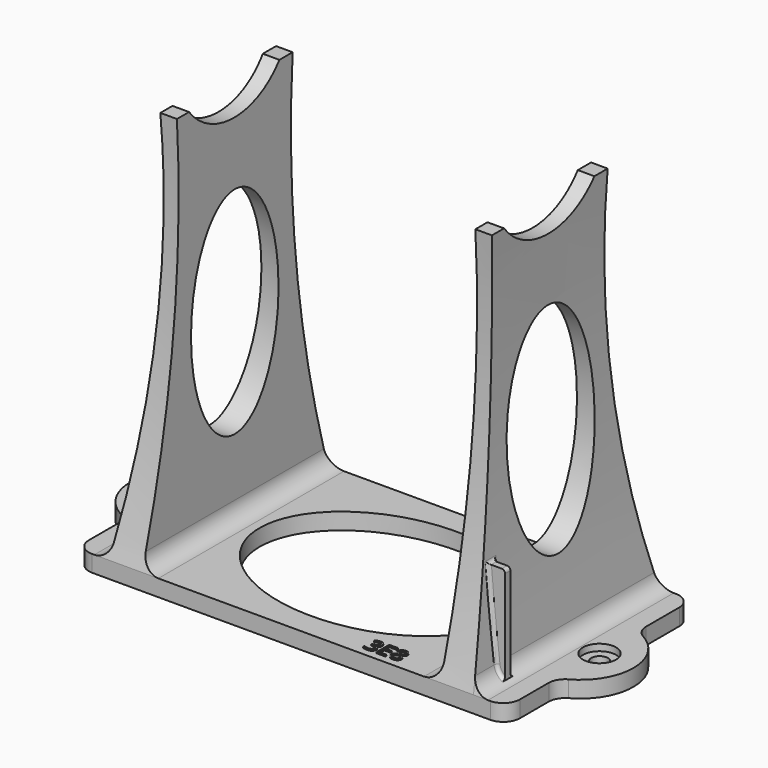
from build123d import *

# Parameters (mm, degrees)
F1_DEPTH       = 35
F3_DEPTH       = 65.001
F3_DEPTH_BACK  = 65.001
F5_DEPTH       = 5.001
F6_DEPTH       = 5
F7_D           = 5
F7_CBORE_D     = 10
F7_CBORE_DEPTH = 2
F8_T1_DEPTH    = 5
F8_T6_DEPTH    = 70
F8_S7_R        = 330
F8_T8_DEPTH    = 37
F8_S9_R        = 330
F8_T10_DEPTH   = 37
F8_T14_DEPTH   = 70
F8_S15_R       = 330
F8_T16_DEPTH   = 37
F8_S17_R       = 330
F8_T18_DEPTH   = 37
F8_T22_DEPTH   = 70
F8_S23_R       = 330
F8_T24_DEPTH   = 37
F8_S25_R       = 330
F8_T26_DEPTH   = 37
F8_T30_DEPTH   = 70
F8_S31_R       = 330
F8_T32_DEPTH   = 37
F8_S33_R       = 330
F8_T34_DEPTH   = 37
F8_T35_DEPTH   = 30.0048285071
F9_TEXT_SIZE   = 6.7275793602
F10_DEPTH      = 0.3
F12_W          = 2
F12_H          = 30
F13_DEPTH      = 5.5
F14_R          = 1


# Not quite as in the source:
# - a fillet or chamfer that OpenCascade refuses, or shapes differently, is made with other operations: its cross-section is extruded or revolved along the edge and cut away or added
# - Text() gives the source's letters only with a copy of the font that has no kerning and outlines rounded to 1/6400 em; it was checked with that copy


with BuildPart() as f1:
    # F0 (on Front) → F1 (new body, symmetric)
    with BuildSketch(Plane.XZ):
        with BuildLine():
            Line((-65, 5), (-65, 0))
            Line((-65, 0), (65, 0))
            Line((65, 0), (65, 5))
            Line((65, 5), (55, 5))
            ThreePointArc((55, 5), (50.1321532001, 62.3970501391), (50, 120))
            Line((50, 120), (45, 120))
            Line((45, 120), (45, 5))
            Line((45, 5), (0, 5))
            Line((0, 5), (-45, 5))
            Line((-45, 5), (-45, 120))
            Line((-45, 120), (-50, 120))
            ThreePointArc((-50, 120), (-50.1321532001, 62.3970501391), (-55, 5))
            Line((-55, 5), (-65, 5))
        make_face()
    extrude(amount=F1_DEPTH, both=True)

    # F2 (on Right) → F3 (cut, two sides)
    with BuildSketch(Plane.YZ) as f3_sk:
        with BuildLine():
            Line((21.2042803188, 133.2788269271), (-21.6306972347, 132.7176760803))
            ThreePointArc((-21.6306972347, 132.7176760803), (-6.9407226467, 112.6628611482), (16.8112740868, 120))
            ThreePointArc((16.8112740868, 120), (20.1221818976, 126.270737315), (21.2042803188, 133.2788269271))
        make_face()
        with BuildLine():
            Line((35, 120), (21.8112740868, 120))
            ThreePointArc((21.8112740868, 120), (23.3239482349, 61.9172086881), (35, 5))
            Line((35, 5), (35, 120))
        make_face()
        with BuildLine():
            add(Edge.make_bspline(
                [(0, 92.5), (-28.5788383249, 92.5), (-14.2894191624, 43.75), (0, -5), (14.2894191624, 43.75), (28.5788383249, 92.5), (0, 92.5)],
                knots=[0, 0, 0, 2.0943951024, 2.0943951024, 4.1887902048, 4.1887902048, 6.2831853072, 6.2831853072, 6.2831853072], degree=2, weights=[1, 0.5, 1, 0.5, 1, 0.5, 1]))
        make_face()
        with BuildLine():
            ThreePointArc((-35, 5), (-23.3239482349, 61.9172086881), (-21.8112740868, 120))
            Line((-21.8112740868, 120), (-35, 120))
            Line((-35, 120), (-35, 5))
        make_face()
    extrude(amount=-F3_DEPTH, mode=Mode.SUBTRACT)
    extrude(f3_sk.sketch, amount=F3_DEPTH_BACK, mode=Mode.SUBTRACT)

    # F4 (on face) → F5 (cut, through all)
    with BuildSketch(Plane.XY.offset(5)):
        with BuildLine():
            add(Edge.make_bspline(
                [(37.5, 0), (37.5, 47.6313972081), (-18.75, 23.8156986041), (-75, 0), (-18.75, -23.8156986041), (37.5, -47.6313972081), (37.5, 0)],
                knots=[0, 0, 0, 2.0943951024, 2.0943951024, 4.1887902048, 4.1887902048, 6.2831853072, 6.2831853072, 6.2831853072], degree=2, weights=[1, 0.5, 1, 0.5, 1, 0.5, 1]))
        make_face()
    extrude(amount=-F5_DEPTH, mode=Mode.SUBTRACT)

    # F4 (on face) → F6 (join)
    with BuildSketch(Plane.XY.offset(5)):
        with BuildLine():
            Line((65, 14.3543907626), (65, -15.9574002028))
            ThreePointArc((65, -15.9574002028), (75.8717613044, -0.8015047201), (65, 14.3543907626))
        make_face()
        with BuildLine():
            ThreePointArc((-65, 14.3543907626), (-75.8717613044, -0.8015047201), (-65, -15.9574002028))
            Line((-65, -15.9574002028), (-65, 14.3543907626))
        make_face()
    extrude(amount=-F6_DEPTH)

    # F7 (through all)
    with Locations(Plane.XY.offset(5)):
        with Locations((65, 0), (-65, -0.8015047201)):
            CounterBoreHole(F7_D / 2, F7_CBORE_D / 2, F7_CBORE_DEPTH)

    # F8: fillet of radius 5 on 12 edges, made by hand

    # F8_s2 → F8_t1 (join)
    with BuildSketch(Plane.XY):
        with BuildLine():
            ThreePointArc((64.9996, -19.1986916005), (65.6953355382, -16.6538385791), (67.58900558, -14.8169012878))
            Line((67.58900558, -14.8169012878), (67.3477327338, -14.3787222566))
            ThreePointArc((67.3477327338, -14.3787222566), (66.118244301, -14.9868786908), (64.8396741415, -15.4835763232))
            Line((64.8396741415, -15.4835763232), (64.4997865958, -15.9574002028))
            ThreePointArc((64.4997865958, -15.9574002028), (64.4997865958, -17.5780459016), (64.4993865958, -19.1986916005))
            Line((64.4993865958, -19.1986916005), (64.9996, -19.1986916005))
        make_face()
        with BuildLine():
            ThreePointArc((-67.58900558, -14.8169012878), (-65.6953355382, -16.6538385791), (-64.9996, -19.1986916005))
            Line((-64.9996, -19.1986916005), (-64.4993865958, -19.1986916005))
            ThreePointArc((-64.4993865958, -19.1986916005), (-64.4997865958, -17.5780459016), (-64.4997865958, -15.9574002028))
            Line((-64.4997865958, -15.9574002028), (-64.8396741415, -15.4835763232))
            ThreePointArc((-64.8396741415, -15.4835763232), (-66.118244301, -14.9868786908), (-67.3477327338, -14.3787222566))
            Line((-67.3477327338, -14.3787222566), (-67.58900558, -14.8169012878))
        make_face()
        with BuildLine():
            ThreePointArc((-64.9996, 17.5956821603), (-65.6953355382, 15.0508291389), (-67.58900558, 13.2138918476))
            Line((-67.58900558, 13.2138918476), (-67.3477327338, 12.7757128164))
            ThreePointArc((-67.3477327338, 12.7757128164), (-66.118244301, 13.3838692506), (-64.8396741415, 13.880566883))
            Line((-64.8396741415, 13.880566883), (-64.4997865958, 14.3543907626))
            ThreePointArc((-64.4997865958, 14.3543907626), (-64.4997865958, 15.9750364614), (-64.4993865958, 17.5956821603))
            Line((-64.4993865958, 17.5956821603), (-64.9996, 17.5956821603))
        make_face()
        with BuildLine():
            ThreePointArc((64.9996, 17.5956821603), (65.6953355382, 15.0508291389), (67.58900558, 13.2138918476))
            Line((67.58900558, 13.2138918476), (67.3477327338, 12.7757128164))
            ThreePointArc((67.3477327338, 12.7757128164), (66.118244301, 13.3838692506), (64.8396741415, 13.880566883))
            Line((64.8396741415, 13.880566883), (64.4997865958, 14.3543907626))
            ThreePointArc((64.4997865958, 14.3543907626), (64.4997865958, 15.9750364614), (64.4993865958, 17.5956821603))
            Line((64.4993865958, 17.5956821603), (64.9996, 17.5956821603))
        make_face()
    extrude(amount=F8_T1_DEPTH)


with BuildPart() as f8_tool4:
    # F8_s5 → F8_t6 (new body)
    with BuildSketch(Plane.XZ.offset(-35)):
        with BuildLine():
            ThreePointArc((59.4227881967, 4.9996), (56.1034800472, 6.2597833835), (54.4568111339, 9.4053119944))
            Line((54.4568111339, 9.4053119944), (53.9602134276, 9.3457231014))
            ThreePointArc((53.9602134276, 9.3457231014), (54.2287059943, 7.1410871793), (54.5037901262, 4.937263414))
            Line((54.5037901262, 4.937263414), (55, 4.4998399076))
            ThreePointArc((55, 4.4998399076), (57.2113940983, 4.4998399076), (59.4227881967, 4.4994399076))
            Line((59.4227881967, 4.4994399076), (59.4227881967, 4.9996))
        make_face()
    extrude(amount=F8_T6_DEPTH)

    # F8_s7 → F8_t8 (cut, symmetric)
    with BuildSketch(Plane.YZ.offset(56.7)):
        with Locations((351.1749527639, 99.5166612019)):
            Circle(F8_S7_R)
    extrude(amount=F8_T8_DEPTH, both=True, mode=Mode.SUBTRACT)

    # F8_s9 → F8_t10 (cut, symmetric)
    with BuildSketch(Plane.YZ.offset(56.7)):
        with Locations((-351.1749527639, 99.5166612019)):
            Circle(F8_S9_R)
    extrude(amount=F8_T10_DEPTH, both=True, mode=Mode.SUBTRACT)


with BuildPart() as f1_1:
    add(f1.part)

    # F8_t3: union F8_tool4
    add(f8_tool4.part)


with BuildPart() as f8_tool12:
    # F8_s13 → F8_t14 (new body)
    with BuildSketch(Plane.XZ.offset(35)):
        with BuildLine():
            ThreePointArc((-59.4227881967, 4.9996), (-56.1034800472, 6.2597833835), (-54.4568111339, 9.4053119944))
            Line((-54.4568111339, 9.4053119944), (-53.9602134276, 9.3457231014))
            ThreePointArc((-53.9602134276, 9.3457231014), (-54.2287059943, 7.1410871793), (-54.5037901262, 4.937263414))
            Line((-54.5037901262, 4.937263414), (-55, 4.4998399076))
            ThreePointArc((-55, 4.4998399076), (-57.2113940983, 4.4998399076), (-59.4227881967, 4.4994399076))
            Line((-59.4227881967, 4.4994399076), (-59.4227881967, 4.9996))
        make_face()
    extrude(amount=-F8_T14_DEPTH)

    # F8_s15 → F8_t16 (cut, symmetric)
    with BuildSketch(Plane.YZ.offset(-56.7)):
        with Locations((351.1749527639, 99.5166612019)):
            Circle(F8_S15_R)
    extrude(amount=F8_T16_DEPTH, both=True, mode=Mode.SUBTRACT)

    # F8_s17 → F8_t18 (cut, symmetric)
    with BuildSketch(Plane.YZ.offset(-56.7)):
        with Locations((-351.1749527639, 99.5166612019)):
            Circle(F8_S17_R)
    extrude(amount=F8_T18_DEPTH, both=True, mode=Mode.SUBTRACT)


with BuildPart() as f1_2:
    add(f1_1.part)

    # F8_t11: union F8_tool12
    add(f8_tool12.part)


with BuildPart() as f8_tool20:
    # F8_s21 → F8_t22 (new body)
    with BuildSketch(Plane.XZ.offset(-35)):
        with BuildLine():
            ThreePointArc((39.9990343146, 4.9996), (43.5355339059, 6.4644660941), (45.0004, 10.0009656854))
            Line((45.0004, 10.0009656854), (45.5005365685, 10.0009656854))
            ThreePointArc((45.5005365685, 10.0009656854), (45.5001365685, 7.5004828427), (45.5001365685, 5))
            Line((45.5001365685, 5), (45, 4.4998634315))
            ThreePointArc((45, 4.4998634315), (42.4995171573, 4.4998634315), (39.9990343146, 4.4994634315))
            Line((39.9990343146, 4.4994634315), (39.9990343146, 4.9996))
        make_face()
    extrude(amount=F8_T22_DEPTH)

    # F8_s23 → F8_t24 (cut, symmetric)
    with BuildSketch(Plane.YZ.offset(42.7)):
        with Locations((351.1749527639, 99.5166612019)):
            Circle(F8_S23_R)
    extrude(amount=F8_T24_DEPTH, both=True, mode=Mode.SUBTRACT)

    # F8_s25 → F8_t26 (cut, symmetric)
    with BuildSketch(Plane.YZ.offset(42.7)):
        with Locations((-351.1749527639, 99.5166612019)):
            Circle(F8_S25_R)
    extrude(amount=F8_T26_DEPTH, both=True, mode=Mode.SUBTRACT)


with BuildPart() as f1_3:
    add(f1_2.part)

    # F8_t19: union F8_tool20
    add(f8_tool20.part)


with BuildPart() as f8_tool28:
    # F8_s29 → F8_t30 (new body)
    with BuildSketch(Plane.XZ.offset(-35)):
        with BuildLine():
            ThreePointArc((-39.9990343146, 4.9996), (-43.5355339059, 6.4644660941), (-45.0004, 10.0009656854))
            Line((-45.0004, 10.0009656854), (-45.5005365685, 10.0009656854))
            ThreePointArc((-45.5005365685, 10.0009656854), (-45.5001365685, 7.5004828427), (-45.5001365685, 5))
            Line((-45.5001365685, 5), (-45, 4.4998634315))
            ThreePointArc((-45, 4.4998634315), (-42.4995171573, 4.4998634315), (-39.9990343146, 4.4994634315))
            Line((-39.9990343146, 4.4994634315), (-39.9990343146, 4.9996))
        make_face()
    extrude(amount=F8_T30_DEPTH)

    # F8_s31 → F8_t32 (cut, symmetric)
    with BuildSketch(Plane.YZ.offset(-42.7)):
        with Locations((351.1749527639, 99.5166612019)):
            Circle(F8_S31_R)
    extrude(amount=F8_T32_DEPTH, both=True, mode=Mode.SUBTRACT)

    # F8_s33 → F8_t34 (cut, symmetric)
    with BuildSketch(Plane.YZ.offset(-42.7)):
        with Locations((-351.1749527639, 99.5166612019)):
            Circle(F8_S33_R)
    extrude(amount=F8_T34_DEPTH, both=True, mode=Mode.SUBTRACT)


with BuildPart() as f1_4:
    add(f1_3.part)

    # F8_t27: union F8_tool28
    add(f8_tool28.part)

    # F8_s36 → F8_t35 (cut)
    with BuildSketch(Plane.XY.offset(-12.5024142536)):
        with BuildLine():
            ThreePointArc((59.9990343146, 35.0004), (63.5355339059, 33.5355339059), (65.0004, 29.9990343146))
            Line((65.0004, 29.9990343146), (65.5005365685, 29.9990343146))
            ThreePointArc((65.5005365685, 29.9990343146), (65.5001365685, 32.4995171573), (65.5001365685, 35))
            Line((65.5001365685, 35), (65, 35.5001365685))
            ThreePointArc((65, 35.5001365685), (62.4995171573, 35.5001365685), (59.9990343146, 35.5005365685))
            Line((59.9990343146, 35.5005365685), (59.9990343146, 35.0004))
        make_face()
        with BuildLine():
            ThreePointArc((-59.9990343146, 35.0004), (-63.5355339059, 33.5355339059), (-65.0004, 29.9990343146))
            Line((-65.0004, 29.9990343146), (-65.5005365685, 29.9990343146))
            ThreePointArc((-65.5005365685, 29.9990343146), (-65.5001365685, 32.4995171573), (-65.5001365685, 35))
            Line((-65.5001365685, 35), (-65, 35.5001365685))
            ThreePointArc((-65, 35.5001365685), (-62.4995171573, 35.5001365685), (-59.9990343146, 35.5005365685))
            Line((-59.9990343146, 35.5005365685), (-59.9990343146, 35.0004))
        make_face()
        with BuildLine():
            ThreePointArc((-59.9990343146, -35.0004), (-63.5355339059, -33.5355339059), (-65.0004, -29.9990343146))
            Line((-65.0004, -29.9990343146), (-65.5005365685, -29.9990343146))
            ThreePointArc((-65.5005365685, -29.9990343146), (-65.5001365685, -32.4995171573), (-65.5001365685, -35))
            Line((-65.5001365685, -35), (-65, -35.5001365685))
            ThreePointArc((-65, -35.5001365685), (-62.4995171573, -35.5001365685), (-59.9990343146, -35.5005365685))
            Line((-59.9990343146, -35.5005365685), (-59.9990343146, -35.0004))
        make_face()
        with BuildLine():
            ThreePointArc((59.9990343146, -35.0004), (63.5355339059, -33.5355339059), (65.0004, -29.9990343146))
            Line((65.0004, -29.9990343146), (65.5005365685, -29.9990343146))
            ThreePointArc((65.5005365685, -29.9990343146), (65.5001365685, -32.4995171573), (65.5001365685, -35))
            Line((65.5001365685, -35), (65, -35.5001365685))
            ThreePointArc((65, -35.5001365685), (62.4995171573, -35.5001365685), (59.9990343146, -35.5005365685))
            Line((59.9990343146, -35.5005365685), (59.9990343146, -35.0004))
        make_face()
    extrude(amount=F8_T35_DEPTH, mode=Mode.SUBTRACT)

    # F9 (on face) → F10 (join)
    with BuildSketch(Plane.XY.offset(5)):
        with Locations((19.3995554, -32.7250659466)):
            Text('3E8', F9_TEXT_SIZE, font='Open Sans', text_align=(TextAlign.LEFT, TextAlign.BOTTOM))
    extrude(amount=F10_DEPTH)

    # F12 (on offset) → F13 (join)
    with BuildSketch(Plane.YZ.offset(57)):
        with Locations((-24.5988334225, 20)):
            Rectangle(F12_W, F12_H)
    extrude(amount=-F13_DEPTH)

    # F14
    f14_edges = [f1_4.edges().sort_by_distance(p)[0] for p in [
        (57, -24.598833, 35),
        (51.862117, -24.598833, 35),
        (53.045276, -25.598833, 22.159178),
        (53.045276, -23.598833, 22.159178),
        (55.290884, -23.598833, 7.1828),
        (55.290884, -25.598833, 7.1828),
    ]]
    fillet(f14_edges, radius=F14_R)


solid = f1_4.part
